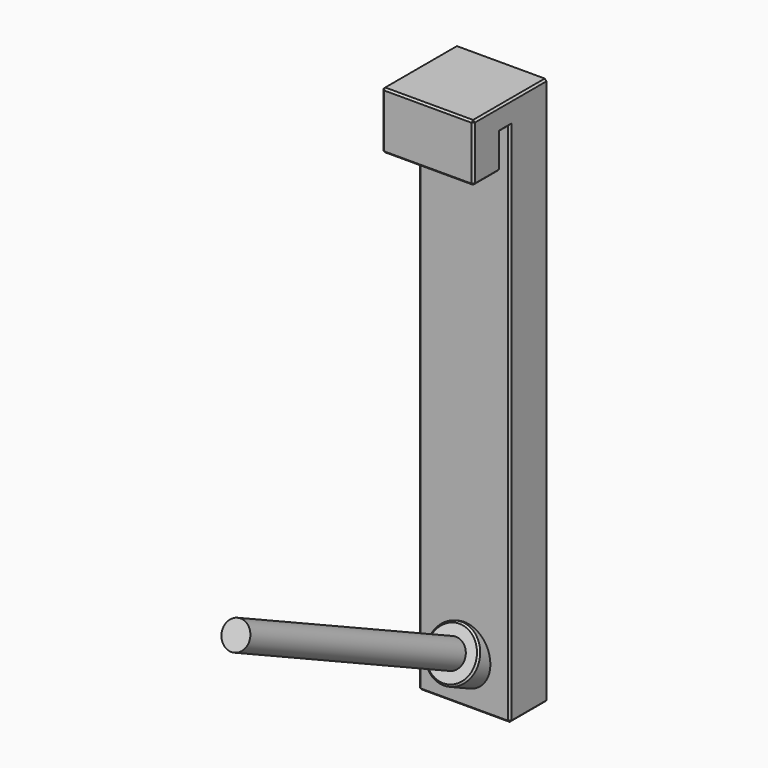
from build123d import *

# Parameters (mm, degrees)
F1_DEPTH = 12.7
F4_SIZE  = 0.5
F6_R     = 7.25
F7_DEPTH = 9.3323626992
F8_SIZE  = 0.5


# Not quite as in the source:
# - a feature names something its author has since deleted; it is built from what else it names


with BuildPart() as f1:
    # F0 (on Right) → F1 (new body, symmetric)
    with BuildSketch(Plane.YZ):
        Polygon((12.7, 76.2), (-12.7, 76.2), (-12.7, 60.325), (-3.302, 60.325), (-3.302, 69.85), (0, 69.85), (0, -76.2), (12.7, -76.2), align=None)
    extrude(amount=F1_DEPTH, both=True)

    # F2 (on Right) → F3 (revolve)
    with BuildSketch(Plane.YZ):
        Polygon((-77.6932350437, -23.067179641), (-79.3034106209, -26.5202123096), (6.35, -66.4610536293), (7.9601755772, -63.0080209607), align=None)
    revolve(axis=Axis((0, -36.4767053105, -46.4906329695), (0, 0.906307787, -0.4226182617)))

    # F4
    f4_edges = [f1.edges().sort_by_distance(p)[0] for p in [
        (-12.7, 0, 76.2),
        (-12.7, 0, -3.175),
        (-12.7, 6.35, -76.2),
        (-12.7, -1.651, 69.85),
        (-12.7, -3.302, 65.0875),
        (-12.7, -12.7, 68.2625),
        (-12.7, -8.001, 60.325),
        (12.7, 6.35, -76.2),
        (12.7, 0, 76.2),
        (12.7, -12.7, 68.2625),
        (12.7, -1.651, 69.85),
        (12.7, -3.302, 65.0875),
        (12.7, -8.001, 60.325),
        (12.7, 0, -3.175),
        (0, 0, -76.2),
        (0, -12.7, 76.2),
        (0, -12.7, 60.325),
        (0, -3.302, 60.325),
    ]]
    chamfer(f4_edges, length=F4_SIZE)

    # F6 (on offset) → F7 (join, up to face)
    with BuildSketch(Plane(origin=(0, 19.834208268, -9.2488432088), x_dir=(1, 0, 0), z_dir=(0, -0.906307787, 0.4226182617))):
        with Locations((0, -57.5505444768)):
            Circle(F6_R)
    extrude(amount=-F7_DEPTH)

    # F8
    f8_edges = [f1.edges().sort_by_distance(p)[0] for p in [
        (-7.25, -4.487703, -61.40735),
    ]]
    chamfer(f8_edges, length=F8_SIZE)


solid = f1.part
